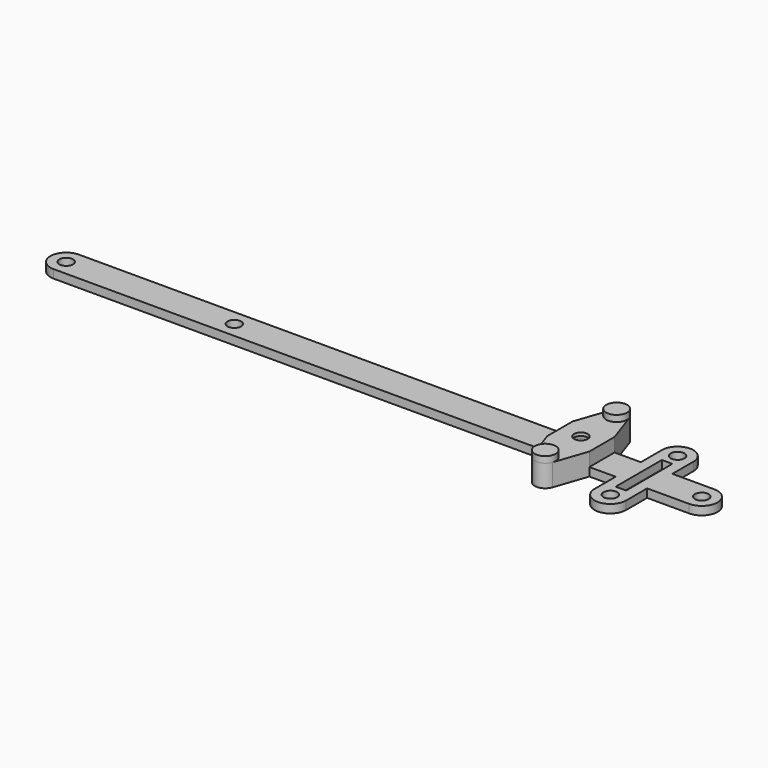
from build123d import *

# Parameters (mm, degrees)
F0_R     = 1.651
F0_W     = 2.54
F0_H     = 13.97
F1_DEPTH = 2.032
F2_R     = 1.651
F3_DEPTH = 3.302
F4_R     = 2.54
F5_DEPTH = 1.524
F6_R     = 2.794
F7_DEPTH = 4.572
F8_R     = 1.14299


# Not quite as in the source:
# - a fillet or chamfer is up to 0.001 mm smaller than in the source, because OpenCascade refuses the exact size


with BuildPart() as f1:
    # F0 (on Top) → F1 (new body)
    with BuildSketch(Plane.XY):
        with BuildLine():
            Line((42.545, 3.81), (-76.835, 3.81))
            ThreePointArc((-76.835, 3.81), (-80.645, 0), (-76.835, -3.81))
            Line((-76.835, -3.81), (42.545, -3.81))
            Line((42.545, -3.81), (45.2222972973, -11.6187837838))
            ThreePointArc((45.2222972973, -11.6187837838), (47.625, -13.335), (50.0277027027, -11.6187837838))
            Line((50.0277027027, -11.6187837838), (52.705, -3.81))
            Line((52.705, -3.81), (59.055, -3.81))
            Line((59.055, -3.81), (59.055, -10.16))
            ThreePointArc((59.055, -10.16), (62.865, -13.97), (66.675, -10.16))
            Line((66.675, -10.16), (66.675, -3.81))
            Line((66.675, -3.81), (76.835, -3.81))
            ThreePointArc((76.835, -3.81), (80.645, 0), (76.835, 3.81))
            Line((76.835, 3.81), (66.675, 3.81))
            Line((66.675, 3.81), (66.675, 10.16))
            ThreePointArc((66.675, 10.16), (62.865, 13.97), (59.055, 10.16))
            Line((59.055, 10.16), (59.055, 3.81))
            Line((59.055, 3.81), (52.705, 3.81))
            Line((52.705, 3.81), (50.0277027027, 11.6187837838))
            ThreePointArc((50.0277027027, 11.6187837838), (47.625, 13.335), (45.2222972973, 11.6187837838))
            Line((45.2222972973, 11.6187837838), (42.545, 3.81))
        make_face()
        with Locations((-76.835, 0)):
            Circle(F0_R, mode=Mode.SUBTRACT)
        with Locations((-36.195, 0)):
            Circle(F0_R, mode=Mode.SUBTRACT)
        with Locations((62.865, -10.16)):
            Circle(F0_R, mode=Mode.SUBTRACT)
        with Locations((47.625, 0)):
            Circle(F0_R, mode=Mode.SUBTRACT)
        with Locations((62.865, 0)):
            Rectangle(F0_W, F0_H, mode=Mode.SUBTRACT)
        with Locations((76.835, 0)):
            Circle(F0_R, mode=Mode.SUBTRACT)
        with Locations((62.865, 10.16)):
            Circle(F0_R, mode=Mode.SUBTRACT)
    extrude(amount=F1_DEPTH)

    # F2 (on face) → F3 (join)
    with BuildSketch(Plane.XY.offset(2.032)):
        with BuildLine():
            ThreePointArc((50.0277027027, 11.6187837838), (47.625, 13.335), (45.2222972973, 11.6187837838))
            Line((45.2222972973, 11.6187837838), (42.545, 3.81))
            Line((42.545, 3.81), (42.545, -3.81))
            Line((42.545, -3.81), (45.2222972973, -11.6187837838))
            ThreePointArc((45.2222972973, -11.6187837838), (47.625, -13.335), (50.0277027027, -11.6187837838))
            Line((50.0277027027, -11.6187837838), (52.705, -3.81))
            Line((52.705, -3.81), (52.705, 3.81))
            Line((52.705, 3.81), (50.0277027027, 11.6187837838))
        make_face()
        with Locations((47.625, 0)):
            Circle(F2_R, mode=Mode.SUBTRACT)
    extrude(amount=F3_DEPTH)

    # F4 (on face) → F5 (join)
    with BuildSketch(Plane.XY.offset(5.334)):
        with Locations((47.625, 10.795)):
            Circle(F4_R)
        with Locations((47.625, -10.795)):
            Circle(F4_R)
    extrude(amount=F5_DEPTH)

    # F6 (on face) → F7 (cut)
    with BuildSketch(Plane(origin=(0, 0, 0), x_dir=(1, 0, 0), z_dir=(0, 0, -1))):
        with Locations((47.625, 0)):
            Circle(F6_R)
    extrude(amount=-F7_DEPTH, mode=Mode.SUBTRACT)

    # F8 (radius 1.143 in the source; OpenCascade refuses exactly that, so slightly less here)
    f8_edges = [f1.edges().sort_by_distance(p)[0] for p in [
        (44.831, 0, 4.572),
    ]]
    fillet(f8_edges, radius=F8_R)


solid = f1.part
